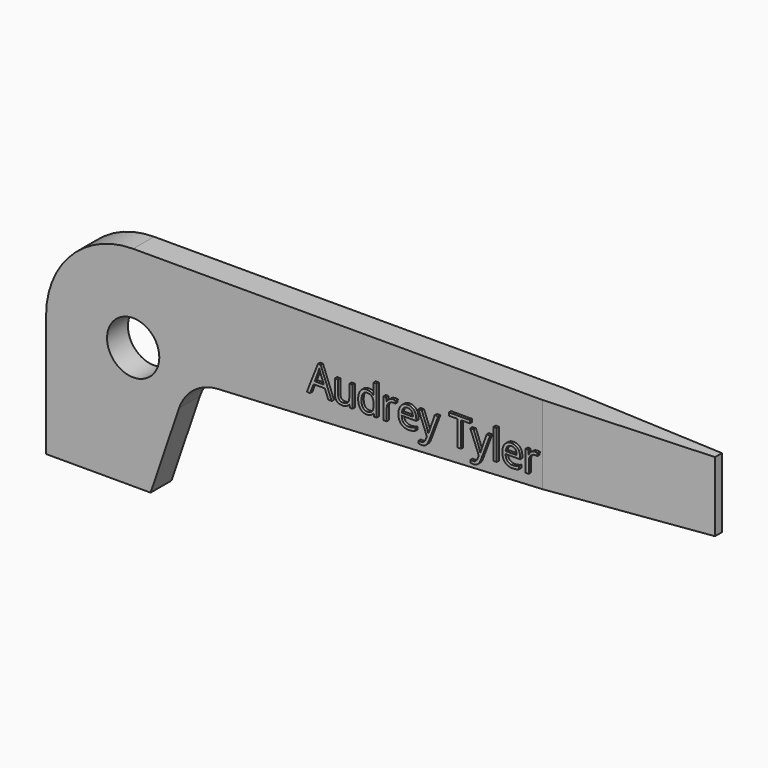
from build123d import *

# Parameters (mm, degrees)
F1_DEPTH     = 2.38125
F2_R         = 2.38125
F3_DEPTH     = 25.4
F5_DEPTH     = 25.4
F6_TEXT_SIZE = 3.5926437277
F7_DEPTH     = 0.254


# Not quite as in the source:
# - Text() gives the source's letters only with a copy of the font that has no kerning and outlines rounded to 1/6400 em; it was checked with that copy


with BuildPart() as f1:
    # F0 (on Front) → F1 (new body)
    with BuildSketch(Plane.XZ):
        with BuildLine():
            Line((60.325, 19.05), (7.9375, 19.05))
            ThreePointArc((7.9375, 19.05), (2.3248399243, 16.7251600757), (0, 11.1125))
            Line((0, 11.1125), (0, 0))
            Line((0, 0), (9.525, 0))
            Line((9.525, 0), (12.1173647876, 7.6271664624))
            ThreePointArc((12.1173647876, 7.6271664624), (13.4786145605, 9.5135918491), (15.6631963617, 10.3130942181))
            Line((15.6631963617, 10.3130942181), (60.325, 12.7))
            Line((60.325, 12.7), (60.325, 19.05))
        make_face()
    extrude(amount=F1_DEPTH)

    # F2 (on face) → F3 (cut)
    with BuildSketch(Plane.XZ.offset(2.38125)):
        with Locations((7.9375, 11.1125)):
            Circle(F2_R)
    extrude(amount=-F3_DEPTH, mode=Mode.SUBTRACT)

    # F4 (on face) → F5 (cut)
    with BuildSketch(Plane.XY.offset(19.05)):
        Polygon((60.325, 0), (45.24375, 0), (60.325, -0.79375), align=None)
        Polygon((60.325, -2.38125), (60.325, -1.5875), (45.24375, -2.38125), align=None)
    extrude(amount=-F5_DEPTH, mode=Mode.SUBTRACT)

    # F6 (on face) → F7 (join)
    with BuildSketch(Plane.XZ.offset(2.38125)):
        with Locations((23.9657561719, 12.8852952947)):
            Text('Audrey Tyler', F6_TEXT_SIZE, font='Open Sans', text_align=(TextAlign.LEFT, TextAlign.BOTTOM))
    extrude(amount=F7_DEPTH)


solid = f1.part
